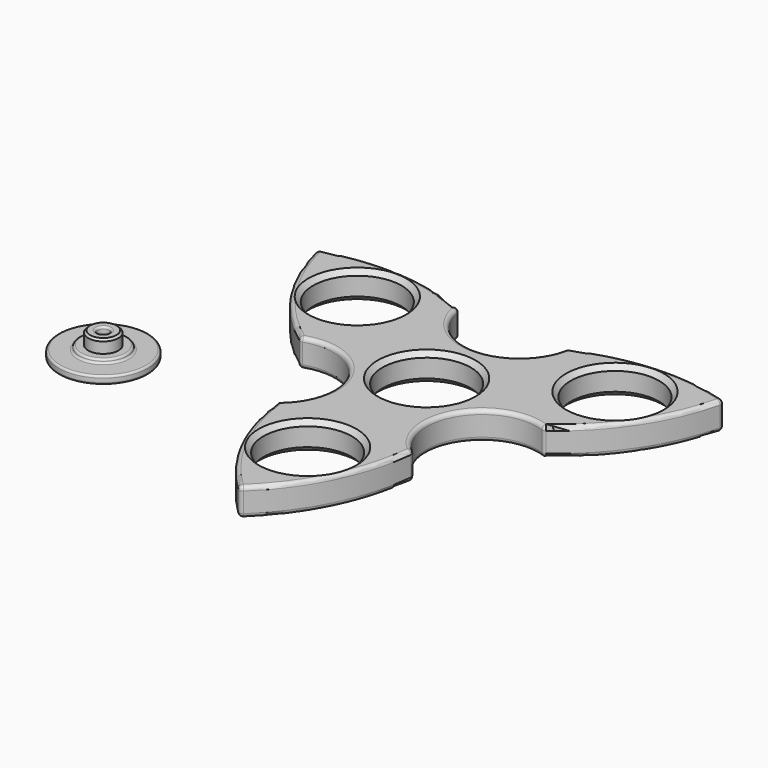
from build123d import *

# Parameters (mm, degrees)
F0_R     = 11.125
F1_DEPTH = 7
F2_R     = 1
F4_R     = 3.8
F4_R_2   = 1.5
F5_DEPTH = 6.25
F4_R_3   = 6.0027241707
F6_DEPTH = 3
F4_R_4   = 11.25
F7_DEPTH = 2
F8_SIZE  = 0.5
F9_R     = 0.49999
F10_R    = 0.5


# Not quite as in the source:
# - a fillet or chamfer that OpenCascade refuses, or shapes differently, is made with other operations: its cross-section is extruded or revolved along the edge and cut away or added
# - a fillet or chamfer is up to 0.001 mm smaller than in the source, because OpenCascade refuses the exact size


with BuildPart() as f1:
    # F0 (on Top) → F1 (new body)
    with BuildSketch(Plane.XY):
        with BuildLine():
            ThreePointArc((-13.9265381796, 27.3563480318), (-32.3399855024, 31.8690177806), (-51.1539637388, 29.5337547347))
            ThreePointArc((-51.1539637388, 29.5337547347), (-43.6607565429, 11.9083607114), (-30.3341287847, -1.8467714635))
            ThreePointArc((-30.3341287847, -1.8467714635), (-13.3225327299, -7.9792749242), (-16.7280232605, -25.7389098662))
            ThreePointArc((-16.7280232605, -25.7389098662), (-11.4293862404, -43.9417578934), (0, -59.0675094694))
            ThreePointArc((0, -59.0675094694), (11.5174353779, -43.7655046703), (16.7664153947, -25.3467403974))
            ThreePointArc((16.7664153947, -25.3467403974), (13.5715211531, -7.5480143247), (30.6545614401, -1.6174381656))
            ThreePointArc((30.6545614401, -1.6174381656), (43.7693717429, 12.0727401128), (51.1539637388, 29.5337547347))
            ThreePointArc((51.1539637388, 29.5337547347), (32.143321165, 31.8571439589), (13.5677133899, 27.193511861))
            ThreePointArc((13.5677133899, 27.193511861), (-0.2489884232, 15.527289249), (-13.9265381796, 27.3563480318))
        make_face()
        with Locations((0, -37.4455563724)):
            Circle(F0_R, mode=Mode.SUBTRACT)
        Circle(F0_R, mode=Mode.SUBTRACT)
        with Locations((-32.4288030773, 18.7227781862)):
            Circle(F0_R, mode=Mode.SUBTRACT)
        with Locations((32.4288030773, 18.7227781862)):
            Circle(F0_R, mode=Mode.SUBTRACT)
    extrude(amount=F1_DEPTH)

    # F2
    f2_edges = [f1.edges().sort_by_distance(p)[0] for p in [
        (-43.660757, 11.908361, 7),
        (-43.660757, 11.908361, 0),
        (-11.429386, -43.941758, 0),
        (-11.429386, -43.941758, 7),
        (-13.322533, -7.979275, 7),
        (-13.322533, -7.979275, 0),
        (-30.334129, -1.846771, 3.5),
        (11.517435, -43.765505, 0),
        (11.517435, -43.765505, 7),
        (16.766415, -25.34674, 3.5),
        (13.571521, -7.548014, 0),
        (13.571521, -7.548014, 7),
        (30.654561, -1.617438, 3.5),
        (43.769372, 12.07274, 7),
        (43.769372, 12.07274, 0),
        (-32.339986, 31.869018, 7),
        (-0.248988, 15.527289, 7),
        (-13.926538, 27.356348, 3.5),
        (32.143321, 31.857144, 7),
        (0, -59.067509, 3.5),
        (51.153964, 29.533755, 3.5),
        (32.143321, 31.857144, 0),
        (13.567713, 27.193512, 3.5),
        (-32.339986, 31.869018, 0),
        (-0.248988, 15.527289, 0),
        (-51.153964, 29.533755, 3.5),
    ]]
    fillet(f2_edges, radius=F2_R)

    # F3: chamfer of 1.2 on 8 edges, made by hand


with BuildPart() as f3_tool1:
    # F3_s2 → F3_t3 (revolve)
    with BuildSketch(Plane.XZ.offset(-18.7227781862)):
        Polygon((-20.1038030773, 7), (-21.3038030773, 5.8), (-21.3038030773, 7), align=None)
    revolve(axis=Axis((-32.4288030773, 18.7227781862, 7), (0, 0, 1)))


with BuildPart() as f3_tool4:
    # F3_s5 → F3_t6 (revolve)
    with BuildSketch(Plane.XZ.offset(-18.7227781862)):
        Polygon((-20.1038030773, 0), (-21.3038030773, 1.2), (-21.3038030773, 0), align=None)
    revolve(axis=Axis((-32.4288030773, 18.7227781862, 0), (0, 0, 1)))


with BuildPart() as f3_tool7:
    # F3_s8 → F3_t9 (revolve)
    with BuildSketch(Plane.XZ.offset(-18.7227781862)):
        Polygon((44.7538030773, 7), (43.5538030773, 5.8), (43.5538030773, 7), align=None)
    revolve(axis=Axis((32.4288030773, 18.7227781862, 7), (0, 0, 1)))


with BuildPart() as f3_tool10:
    # F3_s11 → F3_t12 (revolve)
    with BuildSketch(Plane.XZ.offset(-18.7227781862)):
        Polygon((44.7538030773, 0), (43.5538030773, 1.2), (43.5538030773, 0), align=None)
    revolve(axis=Axis((32.4288030773, 18.7227781862, 0), (0, 0, 1)))


with BuildPart() as f3_tool13:
    # F3_s14 → F3_t15 (revolve)
    with BuildSketch(Plane.XZ.offset(37.4455563724)):
        Polygon((12.325, 7), (11.125, 5.8), (11.125, 7), align=None)
    revolve(axis=Axis((0, -37.4455563724, 7), (0, 0, 1)))


with BuildPart() as f3_tool16:
    # F3_s17 → F3_t18 (revolve)
    with BuildSketch(Plane.XZ.offset(37.4455563724)):
        Polygon((12.325, 0), (11.125, 1.2), (11.125, 0), align=None)
    revolve(axis=Axis((0, -37.4455563724, 0), (0, 0, 1)))


with BuildPart() as f3_tool19:
    # F3_s20 → F3_t21 (revolve)
    with BuildSketch(Plane.XZ):
        Polygon((12.325, 7), (11.125, 5.8), (11.125, 7), align=None)
    revolve(axis=Axis((0, 0, 7), (0, 0, 1)))


with BuildPart() as f3_tool22:
    # F3_s23 → F3_t24 (revolve)
    with BuildSketch(Plane.XZ):
        Polygon((12.325, 0), (11.125, 1.2), (11.125, 0), align=None)
    revolve(axis=Axis((0, 0, 0), (0, 0, 1)))


with BuildPart() as f1_1:
    add(f1.part)

    # F3_t25: cut F3_tool1, F3_tool4, F3_tool7, F3_tool10, F3_tool13, F3_tool16, F3_tool19, F3_tool22
    add([f3_tool1.part, f3_tool4.part, f3_tool7.part, f3_tool10.part, f3_tool13.part, f3_tool16.part, f3_tool19.part, f3_tool22.part], mode=Mode.SUBTRACT)


with BuildPart() as f5:
    # F4 (on Top) → F5 (new body)
    with BuildSketch(Plane.XY):
        with Locations((-63.3144304156, -22.5816704333)):
            Circle(F4_R)
        with Locations((-63.3144304156, -22.5816704333)):
            Circle(F4_R_2, mode=Mode.SUBTRACT)
    extrude(amount=F5_DEPTH)

    # F4 (on Top) → F6 (join)
    with BuildSketch(Plane.XY):
        with Locations((-63.3144304156, -22.5816704333)):
            Circle(F4_R_3)
        with Locations((-63.3144304156, -22.5816704333)):
            Circle(F4_R, mode=Mode.SUBTRACT)
    extrude(amount=F6_DEPTH)

    # F4 (on Top) → F7 (join)
    with BuildSketch(Plane.XY):
        with Locations((-63.3144304156, -22.5816704333)):
            Circle(F4_R_4)
        with Locations((-63.3144304156, -22.5816704333)):
            Circle(F4_R_3, mode=Mode.SUBTRACT)
    extrude(amount=F7_DEPTH)

    # F8
    f8_edges = [f5.edges().sort_by_distance(p)[0] for p in [
        (-67.11443, -22.58167, 6.25),
    ]]
    chamfer(f8_edges, length=F8_SIZE)

    # F9 (radius 0.5 in the source; OpenCascade refuses exactly that, so slightly less here)
    f9_edges = [f5.edges().sort_by_distance(p)[0] for p in [
        (-69.317155, -22.58167, 3),
        (-74.56443, -22.58167, 2),
        (-74.56443, -22.58167, 0),
        (-69.317155, -22.58167, 2),
        (-57.311706, -22.58167, 2.5),
    ]]
    fillet(f9_edges, radius=F9_R)

    # F10
    f10_edges = [f5.edges().sort_by_distance(p)[0] for p in [
        (-64.81443, -22.58167, 0),
        (-61.81443, -22.58167, 3.125),
        (-64.81443, -22.58167, 6.25),
    ]]
    fillet(f10_edges, radius=F10_R)


solid = Compound([f1_1.part, f5.part])
